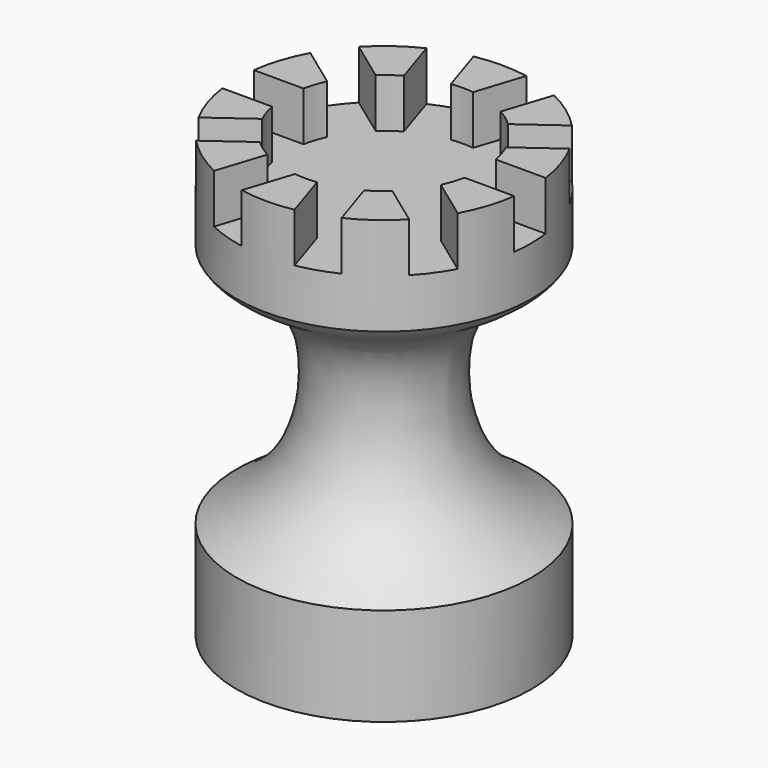
from build123d import *

# Parameters (mm, degrees)
F0_W     = 19.05
F0_H     = 12.7
F2_R     = 12.7
F3_DEPTH = 6.35
F4_W     = 14.3478936436
F4_H     = 5.08
F5_DEPTH = 6.35


# Not quite as in the source:
# - a feature of the source that left no trace in its solid (it failed there, or was rolled back) is left out


with BuildPart() as f1:
    # F0 (on Front) → F1 (revolve)
    with BuildSketch(Plane.XZ):
        with Locations((9.525, 50.8)):
            Rectangle(F0_W, F0_H)
        with BuildLine():
            Line((0, 44.45), (0, 0))
            Line((0, 0), (19.05, 0))
            Line((19.05, 0), (19.05, 12.7))
            add(Edge.make_bspline(
                [(19.05, 12.7), (16.3044854864, 14.4605922783), (11.5816284357, 18.1369797007), (8.0678489786, 26.6218092545), (8.7605074506, 39.8132017689), (17.6573194939, 42.2227860015), (19.05, 44.45)],
                knots=[0, 0, 0, 0, 0.2386598147, 0.4768090303, 0.7479827182, 1, 1, 1, 1], degree=3))
            Line((19.05, 44.45), (0, 44.45))
        make_face()
    revolve(axis=Axis((0, 0, 28.575), (0, 0, 1)))

    # F2 (on face) → F3 (cut)
    with BuildSketch(Plane.XY.offset(57.15)):
        Circle(F2_R)
    extrude(amount=-F3_DEPTH, mode=Mode.SUBTRACT)

    # F4 (on face) → F5 (cut)
    with BuildSketch(Plane.XY.offset(57.15)):
        with Locations((19.05, 0)):
            Rectangle(F4_W, F4_H)
        Polygon((11.1008845043, 4.9257238661), (22.7085742955, 13.3592041513), (19.7226252138, 17.4690104828), (8.1149354226, 9.0355301976), align=None)
        Polygon((6.0855174874, 10.5099886346), (10.5192604568, 24.1556463795), (5.687893354, 25.7254527109), (1.2541503846, 12.079794966), align=None)
        Polygon((-1.2543481381, 12.079794966), (-5.6880911074, 25.7254527109), (-10.5194582102, 24.1556463795), (-6.0857152409, 10.5099886346), align=None)
        Polygon((-8.1151331761, 9.0355301976), (-19.7228229673, 17.4690104828), (-22.7087720489, 13.3592041513), (-11.1010822577, 4.9257238661), align=None)
        with Locations((-19.0501977534, 0)):
            Rectangle(F4_W, F4_H)
        Polygon((-11.1010822577, -4.9257238661), (-22.7087720489, -13.3592041513), (-19.7228229673, -17.4690104828), (-8.1151331761, -9.0355301976), align=None)
        Polygon((-6.0857152409, -10.5099886346), (-10.5194582102, -24.1556463795), (-5.6880911074, -25.7254527109), (-1.2543481381, -12.079794966), align=None)
        Polygon((1.2541503846, -12.079794966), (5.687893354, -25.7254527109), (10.5192604568, -24.1556463795), (6.0855174874, -10.5099886346), align=None)
        Polygon((8.1149354226, -9.0355301976), (19.7226252138, -17.4690104828), (22.7085742955, -13.3592041513), (11.1008845043, -4.9257238661), align=None)
    extrude(amount=-F5_DEPTH, mode=Mode.SUBTRACT)


solid = f1.part
